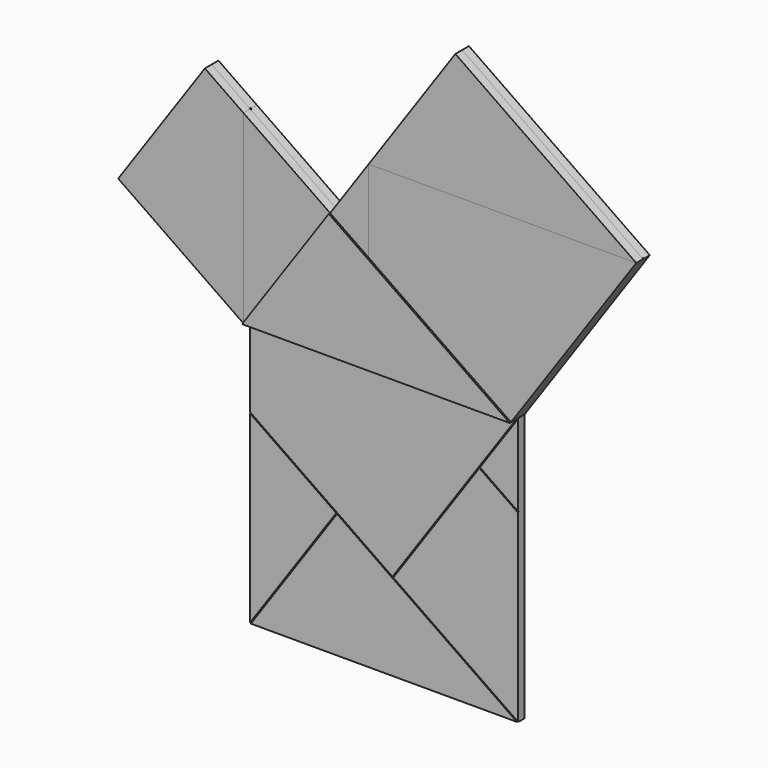
from build123d import *

# Parameters (mm, degrees)
F1_DEPTH = 7.62
F2_DEPTH = 6.35
F3_DEPTH = 6.35
F4_DEPTH = 6.35
F6_DEPTH = 0.762


with BuildPart() as f1:
    # F0 (on Front) → F1 (new body, symmetric)
    with BuildSketch(Plane.XZ):
        Polygon((28.9158669246, -20.0186771016), (0, 0), (-65.0607005803, -93.9765675049), (135.7439308404, -93.9765675049), align=None)
    extrude(amount=F1_DEPTH, both=True)


with BuildPart() as f2:
    # F0 (on Front) → F2 (new body)
    with BuildSketch(Plane.XZ):
        Polygon((28.9158669246, 41.7673633355), (28.9158669246, -20.0186771016), (135.7439308404, -93.9765675049), (229.7204983453, 41.7673633355), align=None)
    extrude(amount=F2_DEPTH)


with BuildPart() as f2b:
    # F0 (on Front) → F2, piece 2 (new body)
    with BuildSketch(Plane.XZ):
        Polygon((-65.0607005803, -93.9765675049), (0, 0), (-65.0607005803, 45.0420234787), align=None)
    extrude(amount=F2_DEPTH)


with BuildPart() as f3:
    # F0 (on Front) → F3 (new body)
    with BuildSketch(Plane.XZ):
        Polygon((93.9765675049, 135.7439308404), (28.9158669246, 41.7673633355), (229.7204983453, 41.7673633355), align=None)
    extrude(amount=F3_DEPTH)


with BuildPart() as f3b:
    # F0 (on Front) → F3, piece 2 (new body)
    with BuildSketch(Plane.XZ):
        Polygon((-159.0372680852, -28.9158669246), (-65.0607005803, -93.9765675049), (-65.0607005803, 45.0420234787), (-93.9765675049, 65.0607005803), align=None)
    extrude(amount=F3_DEPTH)


with BuildPart() as f3c:
    # F0 (on Front) → F3, piece 3 (new body)
    with BuildSketch(Plane.XZ):
        Polygon((28.9158669246, 41.7673633355), (0, 0), (28.9158669246, -20.0186771016), align=None)
    extrude(amount=F3_DEPTH)


with BuildPart() as f4:
    # F0 (on Front) → F4 (new body)
    with BuildSketch(Plane.XZ):
        Polygon((28.9158669246, -20.0186771016), (0, 0), (-65.0607005803, -93.9765675049), (135.7439308404, -93.9765675049), align=None)
        Polygon((28.9158669246, 41.7673633355), (0, 0), (28.9158669246, -20.0186771016), align=None)
        Polygon((-65.0607005803, -93.9765675049), (0, 0), (-65.0607005803, 45.0420234787), align=None)
        Polygon((135.7439308404, -93.9765675049), (-65.0607005803, -93.9765675049), (-65.0607005803, -155.762607942), (0, -200.8046314207), (41.7673633355, -229.7204983453), (106.8280639158, -135.7439308404), align=None)
        Polygon((-159.0372680852, -28.9158669246), (-65.0607005803, -93.9765675049), (-65.0607005803, 45.0420234787), (-93.9765675049, 65.0607005803), align=None)
        Polygon((28.9158669246, 41.7673633355), (28.9158669246, -20.0186771016), (135.7439308404, -93.9765675049), (229.7204983453, 41.7673633355), align=None)
        Polygon((93.9765675049, 135.7439308404), (28.9158669246, 41.7673633355), (229.7204983453, 41.7673633355), align=None)
        Polygon((135.7439308404, -155.762607942), (135.7439308404, -93.9765675049), (106.8280639158, -135.7439308404), align=None)
        Polygon((0, -200.8046314207), (-65.0607005803, -155.762607942), (-65.0607005803, -294.7811989256), align=None)
        Polygon((135.7439308404, -294.7811989256), (135.7439308404, -155.762607942), (106.8280639158, -135.7439308404), (41.7673633355, -229.7204983453), align=None)
        Polygon((0, -200.8046314207), (-65.0607005803, -294.7811989256), (135.7439308404, -294.7811989256), (41.7673633355, -229.7204983453), align=None)
    extrude(amount=-F4_DEPTH)

    # F5 (on face) → F6 (cut)
    with BuildSketch(Plane.XZ):
        with BuildLine():
            ThreePointArc((-64.8438315784, -155.449352717), (-65.3739558053, -155.5457389401), (-65.2775695822, -156.075863167))
            Line((-65.2775695822, -156.075863167), (-0.530124227, -200.9010176438))
            Line((-0.530124227, -200.9010176438), (-0.313255225, -200.5877624188))
            ThreePointArc((-0.313255225, -200.5877624188), (-0.0681555046, -200.4297770127), (0.2168687468, -200.491376019))
            Line((0.2168687468, -200.491376019), (-64.8438315784, -155.449352717))
        make_face()
        with BuildLine():
            Line((-0.313255225, -200.5877624188), (-0.530124227, -200.9010176438))
            Line((-0.530124227, -200.9010176438), (0.0963862231, -201.3347556476))
            Line((0.0963862231, -201.3347556476), (0.313255225, -201.0215004226))
            ThreePointArc((0.313255225, -201.0215004226), (0.374854408, -200.7364759161), (0.2168687468, -200.491376019))
            ThreePointArc((0.2168687468, -200.491376019), (-0.0681555046, -200.4297770127), (-0.313255225, -200.5877624188))
        make_face()
        with BuildLine():
            Line((0.0963862231, -201.3347556476), (-0.530124227, -200.9010176438))
            Line((-0.530124227, -200.9010176438), (-65.3739558053, -294.5643299236))
            ThreePointArc((-65.3739558053, -294.5643299236), (-65.2775695822, -295.0944541506), (-64.7474453553, -294.9980679275))
            Line((-64.7474453553, -294.9980679275), (0.0963862231, -201.3347556476))
        make_face()
        with BuildLine():
            Line((41.6709771124, -229.1903741183), (0.2168687468, -200.491376019))
            ThreePointArc((0.2168687468, -200.491376019), (0.374854408, -200.7364759161), (0.313255225, -201.0215004226))
            Line((0.313255225, -201.0215004226), (0.0963862231, -201.3347556476))
            Line((0.0963862231, -201.3347556476), (41.5504944163, -230.0337536275))
            ThreePointArc((41.5504944163, -230.0337536275), (41.3925089088, -229.7886537467), (41.4541081105, -229.5036293433))
            Line((41.4541081105, -229.5036293433), (41.6709771124, -229.1903741183))
        make_face()
        with BuildLine():
            Line((106.5148086859, -135.5270618455), (41.6709771124, -229.1903741183))
            Line((41.6709771124, -229.1903741183), (42.2974875625, -229.6241121222))
            Line((42.2974875625, -229.6241121222), (106.9244501389, -136.2740550673))
            Line((106.9244501389, -136.2740550673), (106.6111949139, -136.0571860654))
            ThreePointArc((106.6111949139, -136.0571860654), (106.4532094808, -135.8120861966), (106.5148086859, -135.5270618455))
        make_face()
        with BuildLine():
            Line((42.2974875625, -229.6241121222), (41.6709771124, -229.1903741183))
            Line((41.6709771124, -229.1903741183), (41.4541081105, -229.5036293433))
            ThreePointArc((41.4541081105, -229.5036293433), (41.3925089088, -229.7886537467), (41.5504944163, -230.0337536275))
            ThreePointArc((41.5504944163, -230.0337536275), (41.8355187369, -230.095352772), (42.0806185605, -229.9373673472))
            Line((42.0806185605, -229.9373673472), (42.2974875625, -229.6241121222))
        make_face()
        with BuildLine():
            ThreePointArc((42.0806185605, -229.9373673472), (41.8355187369, -230.095352772), (41.5504944163, -230.0337536275))
            Line((41.5504944163, -230.0337536275), (135.5270618385, -295.0944541506))
            ThreePointArc((135.5270618385, -295.0944541506), (136.0571860654, -294.9980679275), (135.9607998423, -294.4679437006))
            Line((135.9607998423, -294.4679437006), (42.2974875625, -229.6241121222))
            Line((42.2974875625, -229.6241121222), (42.0806185605, -229.9373673472))
        make_face()
        with BuildLine():
            ThreePointArc((107.0449329177, -135.4306756154), (106.7599085596, -135.3690764054), (106.5148086859, -135.5270618455))
            ThreePointArc((106.5148086859, -135.5270618455), (106.4532094808, -135.8120861966), (106.6111949139, -136.0571860654))
            Line((106.6111949139, -136.0571860654), (106.9244501389, -136.2740550673))
            Line((106.9244501389, -136.2740550673), (107.3581881428, -135.6475446173))
            Line((107.3581881428, -135.6475446173), (107.0449329177, -135.4306756154))
        make_face()
        with BuildLine():
            Line((135.4306756154, -93.7596985029), (106.5148086859, -135.5270618455))
            ThreePointArc((106.5148086859, -135.5270618455), (106.7599085596, -135.3690764054), (107.0449329177, -135.4306756154))
            Line((107.0449329177, -135.4306756154), (107.3581881428, -135.6475446173))
            Line((107.3581881428, -135.6475446173), (136.0571860654, -94.1934365068))
            ThreePointArc((136.0571860654, -94.1934365068), (135.9607998423, -93.6633122799), (135.4306756154, -93.7596985029))
        make_face()
        with BuildLine():
            Line((107.3581881428, -135.6475446173), (106.9244501389, -136.2740550673))
            Line((106.9244501389, -136.2740550673), (135.5270618385, -156.075863167))
            ThreePointArc((135.5270618385, -156.075863167), (136.0571860654, -155.979476944), (135.9607998423, -155.449352717))
            Line((135.9607998423, -155.449352717), (107.3581881428, -135.6475446173))
        make_face()
        with BuildLine():
            ThreePointArc((-65.4417005803, -93.9765675049), (-65.0607005803, -94.3575675049), (-64.6797005803, -93.9765675049))
            Line((-64.6797005803, -93.9765675049), (-64.6797005803, 45.0420234787))
            ThreePointArc((-64.6797005803, 45.0420234787), (-65.0607005803, 45.4230234787), (-65.4417005803, 45.0420234787))
            Line((-65.4417005803, 45.0420234787), (-65.4417005803, -93.9765675049))
        make_face()
        with BuildLine():
            ThreePointArc((28.9158669246, 41.3863633355), (28.6464592409, 41.4979556519), (28.5348669246, 41.7673633355))
            Line((28.5348669246, 41.7673633355), (28.5348669246, -20.0186771016))
            ThreePointArc((28.5348669246, -20.0186771016), (28.9158669246, -20.3996771016), (29.2968669246, -20.0186771016))
            Line((29.2968669246, -20.0186771016), (29.2968669246, 41.3863633355))
            Line((29.2968669246, 41.3863633355), (28.9158669246, 41.3863633355))
        make_face()
        with BuildLine():
            ThreePointArc((28.9158669246, 42.1483633355), (28.6464592409, 42.0367710191), (28.5348669246, 41.7673633355))
            ThreePointArc((28.5348669246, 41.7673633355), (28.6464592409, 41.4979556519), (28.9158669246, 41.3863633355))
            Line((28.9158669246, 41.3863633355), (29.2968669246, 41.3863633355))
            Line((29.2968669246, 41.3863633355), (29.2968669246, 41.7673633355))
            ThreePointArc((29.2968669246, 41.7673633355), (29.1852746082, 42.0367710191), (28.9158669246, 42.1483633355))
        make_face()
        with BuildLine():
            Line((229.7204983453, 42.1483633355), (28.9158669246, 42.1483633355))
            ThreePointArc((28.9158669246, 42.1483633355), (29.1852746082, 42.0367710191), (29.2968669246, 41.7673633355))
            Line((29.2968669246, 41.7673633355), (29.2968669246, 41.3863633355))
            Line((29.2968669246, 41.3863633355), (229.7204983453, 41.3863633355))
            ThreePointArc((229.7204983453, 41.3863633355), (230.1014983453, 41.7673633355), (229.7204983453, 42.1483633355))
        make_face()
    extrude(amount=-F6_DEPTH, mode=Mode.SUBTRACT)


solid = Compound([f1.part, f2.part, f2b.part, f3.part, f3b.part, f3c.part, f4.part])
